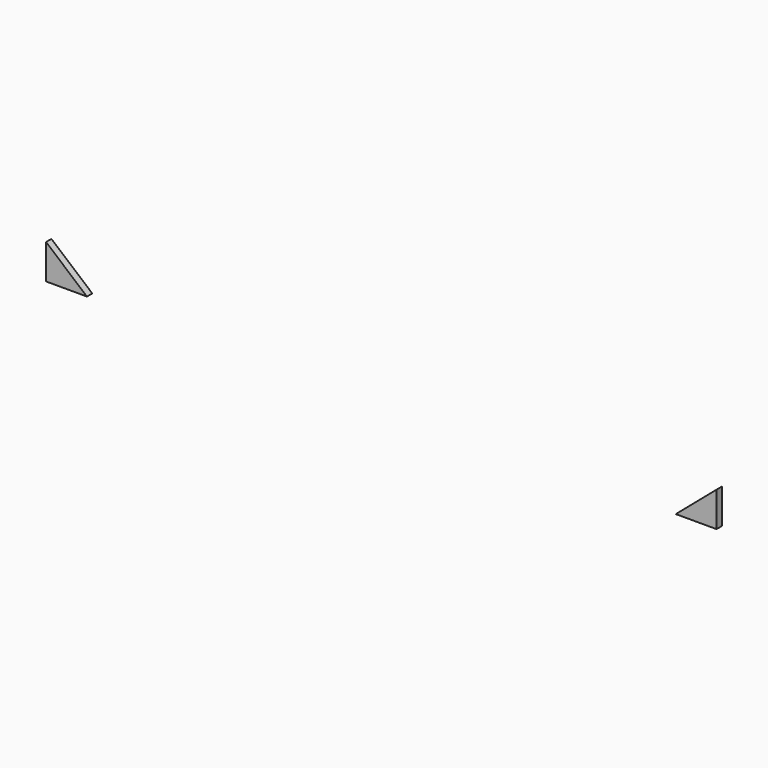
from build123d import *

# Parameters (mm, degrees)
F7_DEPTH = 25.4
F8_DEPTH = 25.4


# Not quite as in the source:
# - the program builds the solid bodies; features that only make, move or delete a surface that nothing else refers to are left out


with BuildPart() as f7:
    # F0 (on Front) → F7 (new body)
    with BuildSketch(Plane.XZ):
        Polygon((1884.7517156601, 0), (1730.0964257692, -131.8028122187), (1884.7517156601, -131.8028122187), align=None)
    extrude(amount=F7_DEPTH)


with BuildPart() as f8:
    # F0 (on Front) → F8 (new body)
    with BuildSketch(Plane.XZ):
        Polygon((-655.2482843399, 0), (-655.2482843399, -131.8028122187), (-500.592994449, -131.8028122187), align=None)
    extrude(amount=F8_DEPTH)


solid = Compound([f7.part, f8.part])
